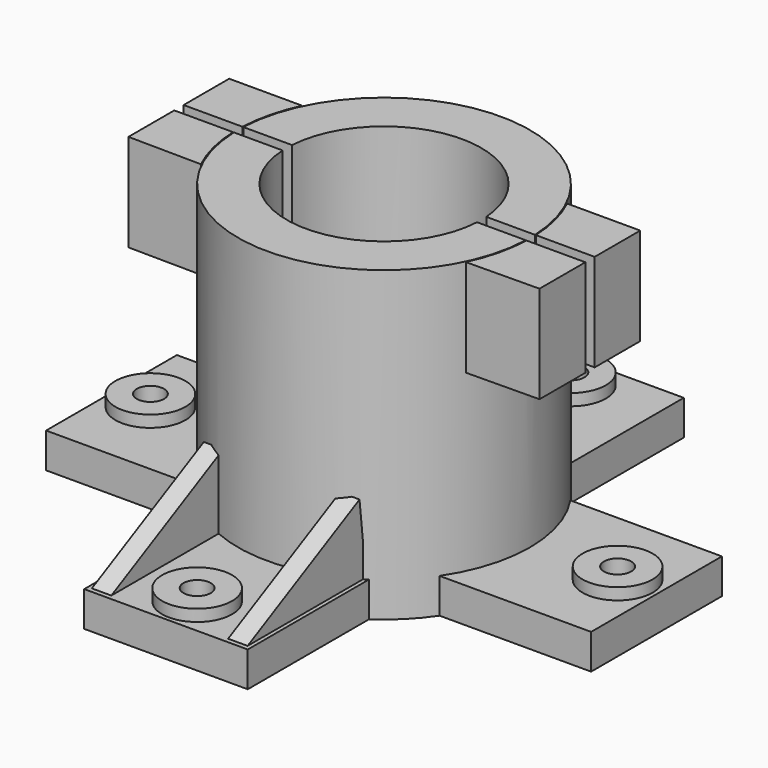
from build123d import *

# Parameters (mm, degrees)
F0_R      = 37.5
F0_R_2    = 25
F1_DEPTH  = 79
F3_DEPTH  = 9
F4_R      = 4
F5_DEPTH  = 10
F6_DEPTH  = 25
F7_R      = 9
F7_R_2    = 3.5
F8_DEPTH  = 12
F12_DEPTH = 25
F9_W      = 3
F9_H      = 35
F13_DEPTH = 70.001
F14_DEPTH = 70.001
F17_DEPTH = 5


# Not quite as in the source:
# - a pattern or mirror of a feature is missing from the dataset's text; its kind, count and spacing are read off the source's solid


with BuildPart() as f1:
    # F0 (on Top) → F1 (new body)
    with BuildSketch(Plane.XY):
        Circle(F0_R)
        Circle(F0_R_2, mode=Mode.SUBTRACT)
    extrude(amount=F1_DEPTH)

    # F2 (on Top) → F3 (join)
    with BuildSketch(Plane.XY):
        with BuildLine():
            Line((-21, 70), (-21, 31.0684727658))
            ThreePointArc((-21, 31.0684727658), (0, 37.5), (21, 31.0684727658))
            Line((21, 31.0684727658), (21, 70))
            Line((21, 70), (-21, 70))
        make_face()
        with BuildLine():
            Line((-70, -21), (-31.0684727658, -21))
            ThreePointArc((-31.0684727658, -21), (-37.5, 0), (-31.0684727658, 21))
            Line((-31.0684727658, 21), (-70, 21))
            Line((-70, 21), (-70, -21))
        make_face()
        with BuildLine():
            Line((21, -70), (21, -31.0684727658))
            ThreePointArc((21, -31.0684727658), (0, -37.5), (-21, -31.0684727658))
            Line((-21, -31.0684727658), (-21, -70))
            Line((-21, -70), (21, -70))
        make_face()
        with BuildLine():
            Line((70, 21), (31.0684727658, 21))
            ThreePointArc((31.0684727658, 21), (37.5, 0), (31.0684727658, -21))
            Line((31.0684727658, -21), (70, -21))
            Line((70, -21), (70, 21))
        make_face()
    extrude(amount=F3_DEPTH)

    # F4 (on Top) → F5 (cut)
    with BuildSketch(Plane.XY):
        with Locations((-60, 0)):
            Circle(F4_R)
        with Locations((0, -60)):
            Circle(F4_R)
        with Locations((60, 0)):
            Circle(F4_R)
        with Locations((0, 60)):
            Circle(F4_R)
    extrude(amount=F5_DEPTH, mode=Mode.SUBTRACT)

    # F4 (on Top) → F6 (cut)
    with BuildSketch(Plane.XY):
        with Locations((-60, 0)):
            Circle(F4_R)
        with Locations((0, -60)):
            Circle(F4_R)
        with Locations((60, 0)):
            Circle(F4_R)
        with Locations((0, 60)):
            Circle(F4_R)
    extrude(amount=F6_DEPTH, mode=Mode.SUBTRACT)

    # F7 (on Top) → F8 (join)
    with BuildSketch(Plane.XY):
        with Locations((-60, 0)):
            Circle(F7_R)
        with Locations((-60, 0)):
            Circle(F7_R_2, mode=Mode.SUBTRACT)
        with Locations((0, -60)):
            Circle(F7_R)
        with Locations((0, -60)):
            Circle(F7_R_2, mode=Mode.SUBTRACT)
        with Locations((60, 0)):
            Circle(F7_R)
        with Locations((60, 0)):
            Circle(F7_R_2, mode=Mode.SUBTRACT)
        with Locations((0, 60)):
            Circle(F7_R)
        with Locations((0, 60)):
            Circle(F7_R_2, mode=Mode.SUBTRACT)
    extrude(amount=F8_DEPTH)


with BuildPart() as f12:
    # F11 (on offset) → F12 (new body)
    with BuildSketch(Plane.XY.offset(79)):
        with BuildLine():
            Line((52.7932941914, 16.2779334933), (34.0223498642, 16.2779334933))
            ThreePointArc((34.0223498642, 16.2779334933), (37.7159304419, 0), (34.0223498642, -16.2779334933))
            Line((34.0223498642, -16.2779334933), (52.7932941914, -16.0596668599))
            Line((52.7932941914, -16.0596668599), (52.7932941914, 16.2779334933))
        make_face()
    extrude(amount=-F12_DEPTH)


with BuildPart() as f12b:
    # F11 (on offset) → F12, piece 2 (new body)
    with BuildSketch(Plane.XY.offset(79)):
        with BuildLine():
            ThreePointArc((-34.0223498642, -16.2779334933), (-37.7159304419, 0), (-34.0223498642, 16.2779334933))
            Line((-34.0223498642, 16.2779334933), (-52.7932941914, 16.2779334933))
            Line((-52.7932941914, 16.2779334933), (-52.7932941914, -16.0596668599))
            Line((-52.7932941914, -16.0596668599), (-34.0223498642, -16.2779334933))
        make_face()
    extrude(amount=-F12_DEPTH)


with BuildPart() as f13_tool:
    # F9 (on Right) → F13 (new body, through all)
    with BuildSketch(Plane.YZ):
        with Locations((0.1505599357, 64.6378623207)):
            Rectangle(F9_W, F9_H)
    extrude(amount=-F13_DEPTH)


with BuildPart() as f1_1:
    add(f1.part)

    # F13: cut by f13_tool
    add(f13_tool.part, mode=Mode.SUBTRACT)


with BuildPart() as f12b_1:
    add(f12b.part)

    # F13: cut by f13_tool
    add(f13_tool.part, mode=Mode.SUBTRACT)


with BuildPart() as f14_tool:
    # F9 (on Right) → F14 (new body, through all)
    with BuildSketch(Plane.YZ):
        with Locations((0.1505599357, 64.6378623207)):
            Rectangle(F9_W, F9_H)
    extrude(amount=F14_DEPTH)


with BuildPart() as f1_2:
    add(f1_1.part)

    # F14: cut by f14_tool
    add(f14_tool.part, mode=Mode.SUBTRACT)

    # F16 (on offset) → F17 (join)
    with BuildSketch(Plane.YZ.offset(15)):
        Polygon((-30.7767703821, 8.7426423561), (-32.8600216546, 27.4980076705), (-69.2997624506, 8.7426423561), align=None)
    f17 = extrude(amount=F17_DEPTH)

    # F17_copies: F17 across plane
    add(f17.mirror(Plane(origin=(0, 0, 0), x_dir=(0, 0, -1), z_dir=(-1, 0, 0))))


with BuildPart() as f12_1:
    add(f12.part)

    # F14: cut by f14_tool
    add(f14_tool.part, mode=Mode.SUBTRACT)


solid = Compound([f12b_1.part, f1_2.part, f12_1.part])
